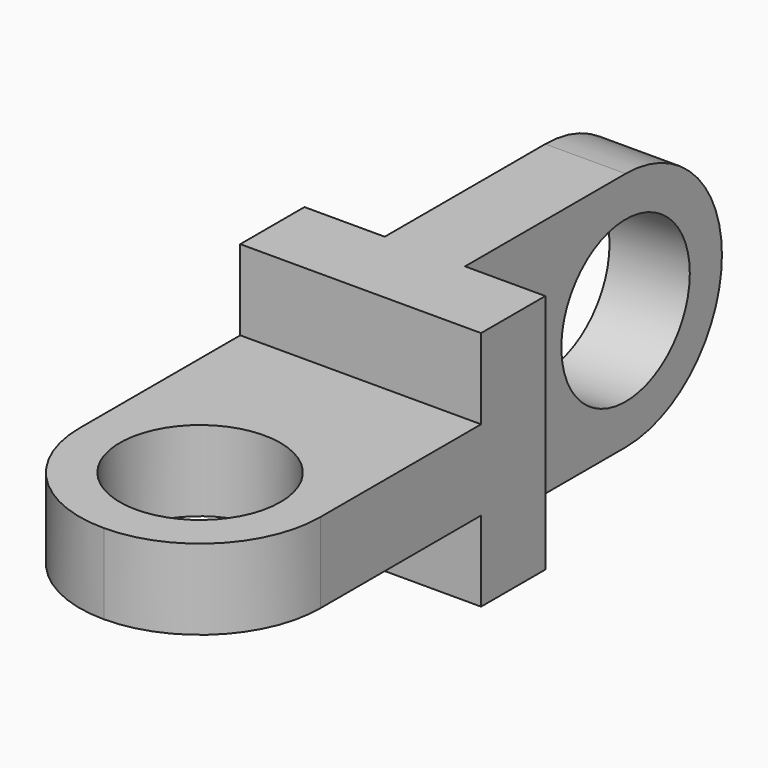
from build123d import *

# Parameters (mm, degrees)
F0_W      = 10
F0_H      = 30
F1_DEPTH  = 15
F2_W      = 30
F2_H      = 10
F3_DEPTH  = 40
F4_R      = 14.99999
F5_W      = 10
F5_H      = 30
F6_DEPTH  = 40
F7_R      = 14.99999
F8_R      = 10
F9_DEPTH  = 10
F10_R     = 10
F11_DEPTH = 10


# Not quite as in the source:
# - a fillet or chamfer is up to 0.001 mm smaller than in the source, because OpenCascade refuses the exact size


with BuildPart() as f1:
    # F0 (on Right) → F1 (new body, symmetric)
    with BuildSketch(Plane.YZ):
        Rectangle(F0_W, F0_H)
    extrude(amount=F1_DEPTH, both=True)

    # F2 (on face) → F3 (join)
    with BuildSketch(Plane.XZ.offset(5)):
        Rectangle(F2_W, F2_H)
    extrude(amount=F3_DEPTH)

    # F4 (radius 15 in the source; OpenCascade refuses exactly that, so slightly less here)
    f4_edges = [f1.edges().sort_by_distance(p)[0] for p in [
        (-15, -45, 0),
        (15, -45, 0),
    ]]
    fillet(f4_edges, radius=F4_R)

    # F5 (on face) → F6 (join)
    with BuildSketch(Plane(origin=(0, 5, 0), x_dir=(-1, 0, 0), z_dir=(0, 1, 0))):
        Rectangle(F5_W, F5_H)
    extrude(amount=F6_DEPTH)

    # F7 (radius 15 in the source; OpenCascade refuses exactly that, so slightly less here)
    f7_edges = [f1.edges().sort_by_distance(p)[0] for p in [
        (0, 45, 15),
        (0, 45, -15),
    ]]
    fillet(f7_edges, radius=F7_R)

    # F8 (on face) → F9 (cut, through all)
    with BuildSketch(Plane.XY.offset(5)):
        with Locations((0, -30)):
            Circle(F8_R)
    extrude(amount=-F9_DEPTH, mode=Mode.SUBTRACT)

    # F10 (on face) → F11 (cut, through all)
    with BuildSketch(Plane.YZ.offset(5)):
        with Locations((30, 0)):
            Circle(F10_R)
    extrude(amount=-F11_DEPTH, mode=Mode.SUBTRACT)


solid = f1.part
